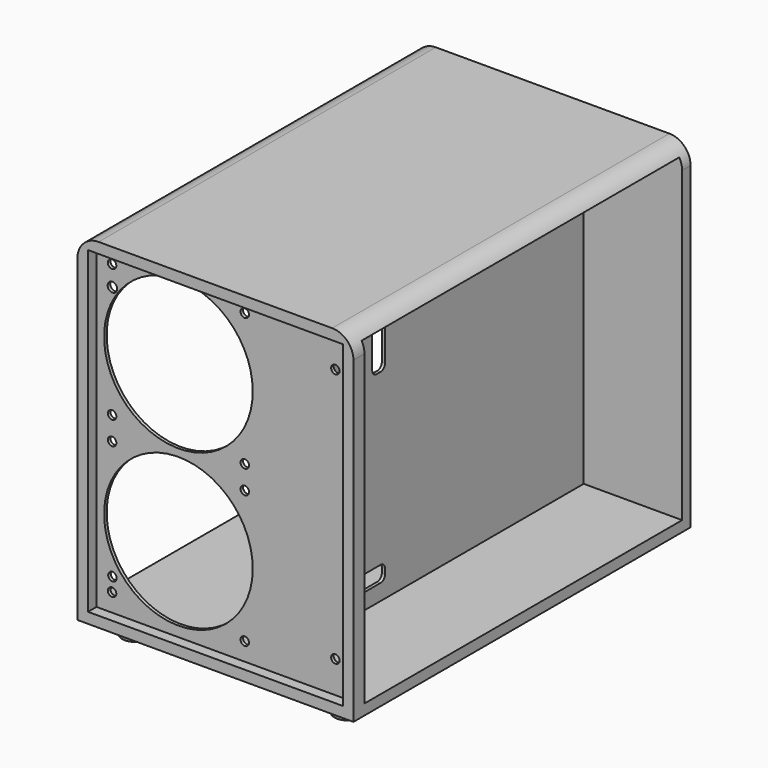
from build123d import *

# Parameters (mm, degrees)
F0_W         = 260
F0_H         = 397
F1_DEPTH     = 320
F2_W         = 240
F2_H         = 300
F3_DEPTH     = 506.73
F5_DEPTH     = 304.8
F6_W         = 3
F6_H         = 377
F7_DEPTH     = 300
F8_R         = 12.5
F9_DEPTH     = 15
F10_R        = 2
F11_W        = 3
F11_H        = 377
F12_DEPTH    = 300
F13_W        = 3
F13_H        = 300
F14_DEPTH    = 87
F15_W        = 3
F15_H        = 300
F16_DEPTH    = 160
F17_R        = 4
F17_R_2      = 70
F18_DEPTH    = 10
F19_W        = 344
F19_H        = 300
F20_DEPTH    = 206
F21_W        = 240
F21_H        = 3
F22_DEPTH    = 300
F23_W        = 44
F23_H        = 159
F23_W_2      = 93.7
F23_H_2      = 15.9
F24_DEPTH    = 25
F25_R        = 4
F25_R_2      = 46
F26_DEPTH    = 25
F27_W        = 3
F27_H        = 300
F28_DEPTH    = 377
F29_W        = 30
F29_H        = 300
F30_DEPTH    = 25
F31_W        = 161.3201568723
F31_H        = 300
F32_DEPTH    = 25
F33_W        = 164.3201568723
F33_H        = 3
F34_DEPTH    = 300
F35_T1_DEPTH = 497
F36_R        = 70
F36_R_2      = 4
F37_DEPTH    = 25
F38_W        = 377
F38_H        = 300
F39_DEPTH    = 3
F40_W        = 5.6798431277
F40_H        = 300
F41_DEPTH    = 3
F42_T1_DEPTH = 497
F43_W        = 3
F43_H        = 374
F44_DEPTH    = 300
F45_W        = 3
F45_H        = 374
F46_DEPTH    = 300
F47_W        = 25
F47_H        = 15
F48_DEPTH    = 25
F49_R        = 5
F51_W        = 15
F51_H        = 40
F51_W_2      = 30
F51_H_2      = 15
F52_DEPTH    = 25
F53_R        = 5
F54_R        = 5
F56_DEPTH    = 25


# Not quite as in the source:
# - a fillet or chamfer that OpenCascade refuses, or shapes differently, is made with other operations: its cross-section is extruded or revolved along the edge and cut away or added


with BuildPart() as f1:
    # F0 (on Top) → F1 (new body)
    with BuildSketch(Plane.XY):
        Rectangle(F0_W, F0_H)
    extrude(amount=F1_DEPTH)

    # F2 (on face) → F3 (cut)
    with BuildSketch(Plane.XZ.offset(198.5)):
        with Locations((0, 160)):
            Rectangle(F2_W, F2_H)
    extrude(amount=-F3_DEPTH, mode=Mode.SUBTRACT)

    # F4 (on face) → F5 (cut)
    with BuildSketch(Plane(origin=(-130, 0, 0), x_dir=(0, -1, 0), z_dir=(-1, 0, 0))):
        Polygon((188.5, 10), (188.5, 310), (-188.5, 310), (-188.5, 10), (0, 10), align=None)
    extrude(amount=-F5_DEPTH, mode=Mode.SUBTRACT)

    # F6 (on face) → F7 (join)
    with BuildSketch(Plane.XY.offset(10)):
        with Locations((-125.8077577353, 0)):
            Rectangle(F6_W, F6_H)
        with Locations((125.8201568723, 0)):
            Rectangle(F6_W, F6_H)
    extrude(amount=F7_DEPTH)

    # F8 (on face) → F9 (join)
    with BuildSketch(Plane(origin=(0, 0, 0), x_dir=(1, 0, 0), z_dir=(0, 0, -1))):
        with Locations((-100, 168.5)):
            Circle(F8_R)
        with Locations((100, 168.5)):
            Circle(F8_R)
        with Locations((100, -168.5)):
            Circle(F8_R)
        with Locations((-100, -168.5)):
            Circle(F8_R)
    extrude(amount=F9_DEPTH)

    # F10
    f10_edges = [f1.edges().sort_by_distance(p)[0] for p in [
        (-112.5, -168.5, -15),
        (87.5, -168.5, -15),
        (87.5, 168.5, -15),
        (-112.5, 168.5, -15),
    ]]
    fillet(f10_edges, radius=F10_R)

    # F11 (on face) → F12 (join)
    with BuildSketch(Plane.XY.offset(10)):
        with Locations((35.8201568723, 0)):
            Rectangle(F11_W, F11_H)
    extrude(amount=F12_DEPTH)

    # F13 (on face) → F14 (join)
    with BuildSketch(Plane.YZ.offset(37.3201568723)):
        with Locations((-187, 160)):
            Rectangle(F13_W, F13_H)
    extrude(amount=F14_DEPTH)

    # F15 (on face) → F16 (join)
    with BuildSketch(Plane(origin=(34.3201568723, 0, 0), x_dir=(0, -1, 0), z_dir=(-1, 0, 0))):
        with Locations((157, 160)):
            Rectangle(F15_W, F15_H)
    extrude(amount=F16_DEPTH)

    # F17 (on face) → F18 (cut)
    with BuildSketch(Plane.XZ.offset(158.5)):
        with Locations((-105.3498431277, 299)):
            Circle(F17_R)
        with Locations((19.6501568723, 299)):
            Circle(F17_R)
        with Locations((-105.3498431277, 174)):
            Circle(F17_R)
        with Locations((19.6501568723, 174)):
            Circle(F17_R)
        with Locations((-42.8498431277, 236.5)):
            Circle(F17_R_2)
        with Locations((-42.8498431277, 83.5)):
            Circle(F17_R_2)
        with Locations((19.6501568723, 146)):
            Circle(F17_R)
        with Locations((19.6501568723, 21)):
            Circle(F17_R)
        with Locations((-105.3498431277, 21)):
            Circle(F17_R)
        with Locations((-105.3498431277, 146)):
            Circle(F17_R)
    extrude(amount=-F18_DEPTH, mode=Mode.SUBTRACT)

    # F19 (on face) → F20 (cut)
    with BuildSketch(Plane.YZ.offset(-124.3077577353)):
        with Locations((16.5, 160)):
            Rectangle(F19_W, F19_H)
    extrude(amount=-F20_DEPTH, mode=Mode.SUBTRACT)

    # F21 (on face) → F22 (join)
    with BuildSketch(Plane.XY.offset(10)):
        with Locations((0, 190)):
            Rectangle(F21_W, F21_H)
    extrude(amount=F22_DEPTH)

    # F23 (on face) → F24 (cut)
    with BuildSketch(Plane.XZ.offset(-188.5)):
        with Locations((4.3201568723, 190.5)):
            Rectangle(F23_W, F23_H)
        with Locations((-30.9022790795, 79.7601031285)):
            Rectangle(F23_W_2, F23_H_2)
        with Locations((-30.8398431277, 98.66)):
            Rectangle(F23_W_2, F23_H_2)
        with Locations((-30.9647150313, 60.8602062571)):
            Rectangle(F23_W_2, F23_H_2)
        with Locations((-31.0271509831, 41.9603093856)):
            Rectangle(F23_W_2, F23_H_2)
    extrude(amount=-F24_DEPTH, mode=Mode.SUBTRACT)

    # F25 (on face) → F26 (cut)
    with BuildSketch(Plane(origin=(0, 191.5, 0), x_dir=(-1, 0, 0), z_dir=(0, 1, 0))):
        with Locations((27.8399215639, 265)):
            Circle(F25_R)
        with Locations((109.8399215639, 265)):
            Circle(F25_R)
        with Locations((27.8399215639, 183)):
            Circle(F25_R)
        with Locations((109.8399215639, 183)):
            Circle(F25_R)
        with Locations((68.8399215639, 224)):
            Circle(F25_R_2)
    extrude(amount=-F26_DEPTH, mode=Mode.SUBTRACT)

    # F27 (on face) → F28 (cut)
    with BuildSketch(Plane.XZ.offset(-188.5)):
        with Locations((-128.5, 160)):
            Rectangle(F27_W, F27_H)
    extrude(amount=F28_DEPTH, mode=Mode.SUBTRACT)

    # F29 (on face) → F30 (cut)
    with BuildSketch(Plane(origin=(-127, 0, 0), x_dir=(0, -1, 0), z_dir=(-1, 0, 0))):
        with Locations((173.5, 160)):
            Rectangle(F29_W, F29_H)
    extrude(amount=-F30_DEPTH, mode=Mode.SUBTRACT)

    # F31 (on face) → F32 (cut)
    with BuildSketch(Plane(origin=(0, -155.5, 0), x_dir=(-1, 0, 0), z_dir=(0, 1, 0))):
        with Locations((46.3399215639, 160)):
            Rectangle(F31_W, F31_H)
    extrude(amount=-F32_DEPTH, mode=Mode.SUBTRACT)

    # F33 (on face) → F34 (join)
    with BuildSketch(Plane.XY.offset(10)):
        with Locations((-47.8399215639, -187)):
            Rectangle(F33_W, F33_H)
    extrude(amount=F34_DEPTH)

    # F35: fillet of radius 20 on 1 edges, made by hand

    # F35_s2 → F35_t1 (cut)
    with BuildSketch(Plane.XZ.offset(-248.5)):
        with BuildLine():
            ThreePointArc((-130, 300), (-124.1421356237, 314.1421356237), (-110, 320))
            Line((-110, 320), (-130, 320))
            Line((-130, 320), (-130, 300))
        make_face()
    extrude(amount=F35_T1_DEPTH, mode=Mode.SUBTRACT)

    # F36 (on face) → F37 (cut)
    with BuildSketch(Plane.XZ.offset(188.5)):
        with Locations((-42.84, 236.5)):
            Circle(F36_R)
        with Locations((-105.34, 299)):
            Circle(F36_R_2)
        with Locations((19.66, 299)):
            Circle(F36_R_2)
        with Locations((-105.34, 174)):
            Circle(F36_R_2)
        with Locations((19.66, 174)):
            Circle(F36_R_2)
        with Locations((-42.84, 89.5)):
            Circle(F36_R)
        with Locations((-105.34, 152)):
            Circle(F36_R_2)
        with Locations((19.66, 152)):
            Circle(F36_R_2)
        with Locations((19.66, 27)):
            Circle(F36_R_2)
        with Locations((-105.34, 27)):
            Circle(F36_R_2)
    extrude(amount=-F37_DEPTH, mode=Mode.SUBTRACT)

    # F38 (on face) → F39 (cut)
    with BuildSketch(Plane.YZ.offset(127.3201568723)):
        with Locations((0, 160)):
            Rectangle(F38_W, F38_H)
    extrude(amount=-F39_DEPTH, mode=Mode.SUBTRACT)

    # F40 (on face) → F41 (join)
    with BuildSketch(Plane(origin=(0, -188.5, 0), x_dir=(-1, 0, 0), z_dir=(0, 1, 0))):
        with Locations((-127.1600784361, 160)):
            Rectangle(F40_W, F40_H)
    extrude(amount=F41_DEPTH)

    # F42: fillet of radius 20 on 1 edges, made by hand

    # F42_s2 → F42_t1 (cut)
    with BuildSketch(Plane.XZ.offset(-248.5)):
        with BuildLine():
            ThreePointArc((110, 320), (124.1421356237, 314.1421356237), (130, 300))
            Line((130, 300), (130, 320))
            Line((130, 320), (110, 320))
        make_face()
    extrude(amount=F42_T1_DEPTH, mode=Mode.SUBTRACT)

    # F47 (on face) → F48 (cut)
    with BuildSketch(Plane(origin=(34.3201568723, 0, 0), x_dir=(0, -1, 0), z_dir=(-1, 0, 0))):
        with Locations((-148.5, 280)):
            Rectangle(F47_W, F47_H)
    extrude(amount=-F48_DEPTH, mode=Mode.SUBTRACT)

    # F49
    f49_edges = [f1.edges().sort_by_distance(p)[0] for p in [
        (35.820157, 161, 272.5),
        (35.820157, 161, 287.5),
        (35.820157, 136, 287.5),
        (35.820157, 136, 272.5),
    ]]
    fillet(f49_edges, radius=F49_R)

    # F51 (on face) → F52 (cut)
    with BuildSketch(Plane.YZ.offset(37.3201568723)):
        with Locations((-53, 220.0625501573)):
            Rectangle(F51_W, F51_H)
        with Locations((-60.5, 32.5625501573)):
            Rectangle(F51_W_2, F51_H_2)
    extrude(amount=-F52_DEPTH, mode=Mode.SUBTRACT)

    # F53
    f53_edges = [f1.edges().sort_by_distance(p)[0] for p in [
        (35.820157, -75.5, 25.06255),
        (35.820157, -75.5, 40.06255),
        (35.820157, -45.5, 25.06255),
        (35.820157, -45.5, 40.06255),
    ]]
    fillet(f53_edges, radius=F53_R)

    # F54
    f54_edges = [f1.edges().sort_by_distance(p)[0] for p in [
        (35.820157, -60.5, 200.06255),
        (35.820157, -45.5, 200.06255),
        (35.820157, -45.5, 240.06255),
        (35.820157, -60.5, 240.06255),
    ]]
    fillet(f54_edges, radius=F54_R)

    # F55 (on face) → F56 (cut)
    with BuildSketch(Plane.XZ.offset(198.5)):
        with BuildLine():
            ThreePointArc((-101, 40), (-105, 44), (-109, 40))
            Line((-109, 40), (-105, 40))
            Line((-105, 40), (-105, 36))
            ThreePointArc((-105, 36), (-102.1715728753, 37.1715728753), (-101, 40))
        make_face()
        with BuildLine():
            Line((-105, 40), (-109, 40))
            ThreePointArc((-109, 40), (-107.8284271247, 37.1715728753), (-105, 36))
            Line((-105, 36), (-105, 40))
        make_face()
        with BuildLine():
            ThreePointArc((105, 36), (107.8284271247, 37.1715728753), (109, 40))
            Line((109, 40), (105, 40))
            Line((105, 40), (105, 36))
        make_face()
        with BuildLine():
            Line((105, 40), (109, 40))
            ThreePointArc((109, 40), (102.1715728753, 42.8284271247), (105, 36))
            Line((105, 36), (105, 40))
        make_face()
        with BuildLine():
            ThreePointArc((105, 284), (102.1715728753, 277.1715728753), (109, 280))
            Line((109, 280), (105, 280))
            Line((105, 280), (105, 284))
        make_face()
        with BuildLine():
            Line((105, 280), (109, 280))
            ThreePointArc((109, 280), (107.8284271247, 282.8284271247), (105, 284))
            Line((105, 284), (105, 280))
        make_face()
        with BuildLine():
            ThreePointArc((-105, 284.5), (-108.1819805153, 283.1819805153), (-109.5, 280))
            Line((-109.5, 280), (-105, 280))
            Line((-105, 280), (-105, 284.5))
        make_face()
        with BuildLine():
            Line((-105, 280), (-109.5, 280))
            ThreePointArc((-109.5, 280), (-105, 275.5), (-100.5, 280))
            ThreePointArc((-100.5, 280), (-101.8180194847, 283.1819805153), (-105, 284.5))
            Line((-105, 284.5), (-105, 280))
        make_face()
    extrude(amount=-F56_DEPTH, mode=Mode.SUBTRACT)


with BuildPart() as f44:
    # F43 (on face) → F44 (new body)
    with BuildSketch(Plane(origin=(0, 0, 310), x_dir=(1, 0, 0), z_dir=(0, 0, -1))):
        with Locations((-125.8205080757, -1.5)):
            Rectangle(F43_W, F43_H)
    extrude(amount=F44_DEPTH)


with BuildPart() as f46:
    # F45 (on face) → F46 (new body)
    with BuildSketch(Plane(origin=(0, 0, 310), x_dir=(1, 0, 0), z_dir=(0, 0, -1))):
        with Locations((125.8205080757, -1.5)):
            Rectangle(F45_W, F45_H)
    extrude(amount=F46_DEPTH)


solid = f1.part
